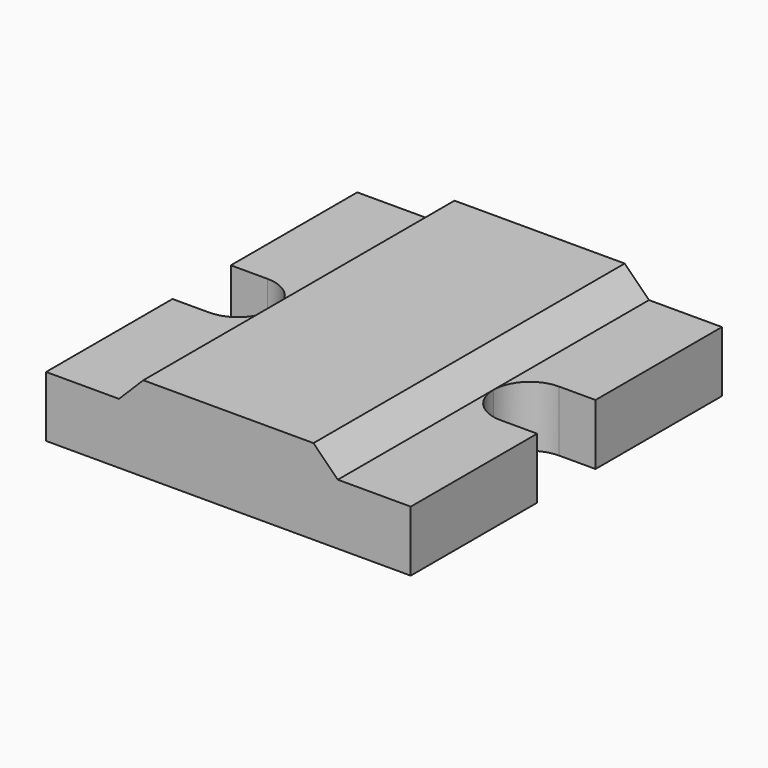
from build123d import *

# Parameters (mm, degrees)
F1_DEPTH = 1.6
F2_W     = 0.3
F2_H     = 0.3
F3_DEPTH = 0.3
F4_W     = 0.3
F4_H     = 0.3
F5_DEPTH = 0.3
F6_R     = 0.14999


# Not quite as in the source:
# - a fillet or chamfer is up to 0.001 mm smaller than in the source, because OpenCascade refuses the exact size


with BuildPart() as f1:
    # F0 (on Front) → F1 (new body)
    with BuildSketch(Plane.XZ):
        Polygon((0.75, -0.125), (0.75, 0.125), (0.45, 0.125), (0.35, 0.225), (-0.35, 0.225), (-0.45, 0.125), (-0.75, 0.125), (-0.75, -0.125), align=None)
    extrude(amount=F1_DEPTH)

    # F2 (on face) → F3 (cut)
    with BuildSketch(Plane.XY.offset(0.125)):
        with Locations((-0.6, -0.8)):
            Rectangle(F2_W, F2_H)
    extrude(amount=-F3_DEPTH, mode=Mode.SUBTRACT)

    # F4 (on face) → F5 (cut)
    with BuildSketch(Plane.XY.offset(0.125)):
        with Locations((0.6, -0.8)):
            Rectangle(F4_W, F4_H)
    extrude(amount=-F5_DEPTH, mode=Mode.SUBTRACT)

    # F6 (radius 0.15 in the source; OpenCascade refuses exactly that, so slightly less here)
    f6_edges = [f1.edges().sort_by_distance(p)[0] for p in [
        (0.45, -0.65, 0),
        (-0.45, -0.65, 0),
        (-0.45, -0.95, 0),
        (0.45, -0.95, 0),
    ]]
    fillet(f6_edges, radius=F6_R)


solid = f1.part
